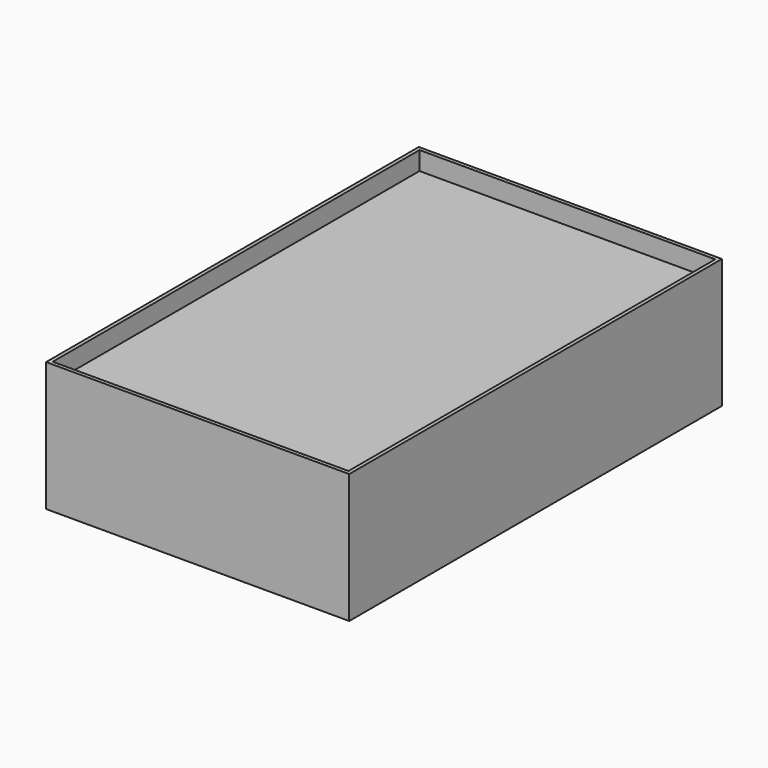
from build123d import *

# Parameters (mm, degrees)
F0_W     = 82
F0_H     = 126
F1_DEPTH = 35
F2_W     = 80
F2_H     = 124
F3_DEPTH = 5
F4_DEPTH = 1
F5_T     = -1
F6_R     = 2.5
F7_DEPTH = 3


with BuildPart() as f1:
    # F0 (on Top) → F1 (new body)
    with BuildSketch(Plane.XY):
        with Locations((-0.2664038911, -0.5331769297)):
            Rectangle(F0_W, F0_H)
    extrude(amount=F1_DEPTH)

    # F2 (on face) → F3 (cut)
    with BuildSketch(Plane.XY.offset(35)):
        with Locations((-0.2664038911, -0.5331769297)):
            Rectangle(F2_W, F2_H)
    extrude(amount=-F3_DEPTH, mode=Mode.SUBTRACT)

    # F4 (add): a face of the model
    f4_faces = [f1.faces().sort_by_distance(p)[0] for p in [
        (-0.2664038911, -0.5331769297, 30),
    ]]
    extrude(f4_faces, amount=-F4_DEPTH)

    # F5 (hollow: no face is removed)
    offset(amount=F5_T, kind=Kind.INTERSECTION, mode=Mode.SUBTRACT)

    # F6 (on face) → F7 (cut)
    with BuildSketch(Plane(origin=(-41.2664038911, 0, 0), x_dir=(0, -1, 0), z_dir=(-1, 0, 0))):
        with Locations((53.5331769297, 7)):
            Circle(F6_R)
    extrude(amount=-F7_DEPTH, mode=Mode.SUBTRACT)


solid = f1.part
